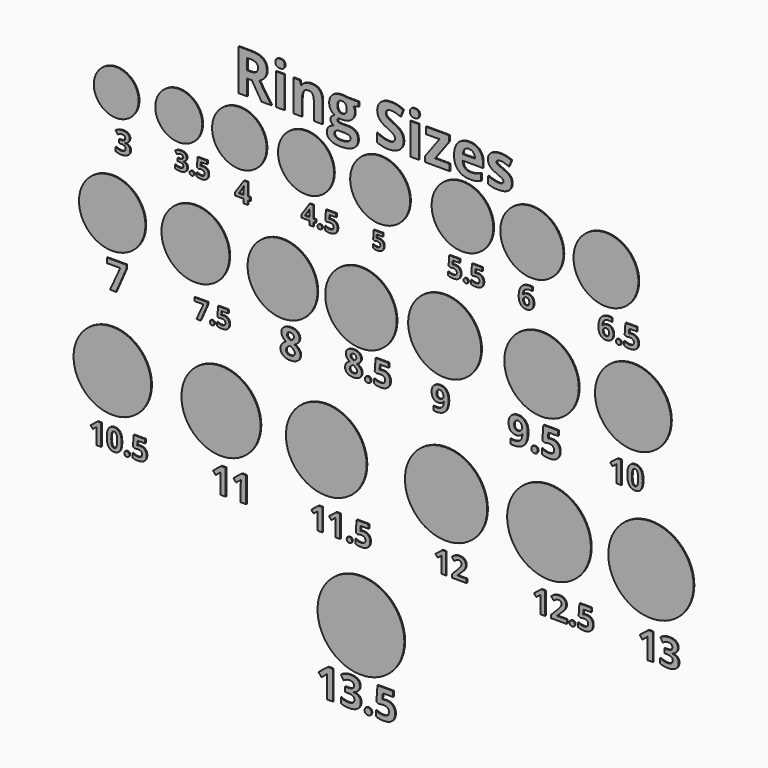
from build123d import *

# Parameters (mm, degrees)
F0_R           = 5.8371680151
F8_DEPTH       = 0.254
F0_R_2         = 6.1199922199
F0_R_3         = 7.0989140275
F0_R_4         = 7.291492477
F0_R_5         = 7.8
F1_R           = 8.0243902439
F1_R_2         = 8.225
F1_R_3         = 8.45
F1_TEXT_SIZE   = 7.715160696
F1_TEXT_SIZE_2 = 6.496977155
F1_TEXT_SIZE_3 = 7.3090960558
F1_TEXT_SIZE_4 = 6.9030366054
F1_TEXT_SIZE_5 = 6.0909125149
F1_TEXT_SIZE_6 = 7.7151555062
F9_DEPTH       = 0.254
F2_R           = 8.65
F2_R_2         = 8.85
F3_R           = 9.1
F3_R_2         = 9.3
F4_R           = 9.504040404
F4_R_2         = 9.7
F4_TEXT_SIZE   = 9.9162159498
F4_TEXT_SIZE_2 = 6.7430258573
F4_TEXT_SIZE_3 = 10.3128641568
F4_TEXT_SIZE_4 = 8.7262694274
F4_TEXT_SIZE_5 = 8.7262713285
F5_R           = 9.9
F5_TEXT_SIZE   = 8.0965381737
F6_R           = 10.1
F6_R_2         = 10.3
F6_R_3         = 10.5
F6_R_4         = 10.7
F6_R_5         = 10.9
F6_R_6         = 11.1
F6_R_7         = 11.3
F6_TEXT_SIZE   = 7.6917129465
F6_TEXT_SIZE_2 = 9.3110190291
F6_TEXT_SIZE_3 = 8.0965355866
F6_TEXT_SIZE_4 = 8.0965407607
F6_TEXT_SIZE_5 = 9.7158468432
F6_TEXT_SIZE_6 = 10.5254921234
F10_DEPTH      = 0.254
F7_TEXT_SIZE   = 14.9785903179
F11_DEPTH      = 0.254


# Not quite as in the source:
# - Text() gives the source's letters only with a copy of the font that has no kerning and outlines rounded to 1/6400 em; it was checked with that copy


with BuildPart() as f8:
    # F0 (on Front) → F8 (new body)
    with BuildSketch(Plane.XZ):
        with Locations((-63.7036129132, 51.7368838191)):
            Circle(F0_R)
    extrude(amount=F8_DEPTH)


with BuildPart() as f8b:
    # F0 (on Front) → F8, piece 2 (new body)
    with BuildSketch(Plane.XZ):
        with Locations((-47.4188692464, 51.7368838191)):
            Circle(F0_R_2)
    extrude(amount=F8_DEPTH)


with BuildPart() as f8c:
    # F0 (on Front) → F8, piece 3 (new body)
    with BuildSketch(Plane.XZ):
        with Locations((-31.6557335996, 51.7368838191)):
            Circle(F0_R_3)
    extrude(amount=F8_DEPTH)


with BuildPart() as f8d:
    # F0 (on Front) → F8, piece 4 (new body)
    with BuildSketch(Plane.XZ):
        with Locations((-14.2972320278, 51.7368838191)):
            Circle(F0_R_4)
    extrude(amount=F8_DEPTH)


with BuildPart() as f8e:
    # F0 (on Front) → F8, piece 5 (new body)
    with BuildSketch(Plane.XZ):
        with Locations((5.0005266884, 51.7368838191)):
            Circle(F0_R_5)
    extrude(amount=F8_DEPTH)


with BuildPart() as f9:
    # F1 (on Front) → F9 (new body)
    with BuildSketch(Plane.XZ):
        with Locations((26.4269726021, 52.6113137603)):
            Circle(F1_R)
        with Locations((44.5094197899, 52.6113137603)):
            Circle(F1_R_2)
        with Locations((63.7865934914, 52.6113137603)):
            Circle(F1_R_3)
        with Locations((-64.1658629432, 37.9931100235)):
            Text('3', F1_TEXT_SIZE, font='Open Sans', font_style=FontStyle.BOLD, text_align=(TextAlign.LEFT, TextAlign.BOTTOM))
        with Locations((-48.670567057, 39.1625649773)):
            Text('3.5', F1_TEXT_SIZE_2, font='Open Sans', font_style=FontStyle.BOLD, text_align=(TextAlign.LEFT, TextAlign.BOTTOM))
        with Locations((-32.8829083665, 37.1160178741)):
            Text('4', F1_TEXT_SIZE_3, font='Open Sans', font_style=FontStyle.BOLD, text_align=(TextAlign.LEFT, TextAlign.BOTTOM))
        with Locations((-15.6334272472, 37.7007472193)):
            Text('4.5', F1_TEXT_SIZE_4, font='Open Sans', font_style=FontStyle.BOLD, text_align=(TextAlign.LEFT, TextAlign.BOTTOM))
        with Locations((2.7855095265, 37.7007472193)):
            Text('5', F1_TEXT_SIZE_5, font='Open Sans', font_style=FontStyle.BOLD, text_align=(TextAlign.LEFT, TextAlign.BOTTOM))
        with Locations((22.3738989185, 37.7007472193)):
            Text('5.5', F1_TEXT_SIZE_4, font='Open Sans', font_style=FontStyle.BOLD, text_align=(TextAlign.LEFT, TextAlign.BOTTOM))
        with Locations((40.7928359258, 36.8236550698)):
            Text('6', F1_TEXT_SIZE_6, font='Open Sans', font_style=FontStyle.BOLD, text_align=(TextAlign.LEFT, TextAlign.BOTTOM))
        with Locations((61.5506847088, 36.5312885289)):
            Text('6.5', F1_TEXT_SIZE, font='Open Sans', font_style=FontStyle.BOLD, text_align=(TextAlign.LEFT, TextAlign.BOTTOM))
    extrude(amount=F9_DEPTH)


with BuildPart() as f10:
    # F2 (on Front) + F3 (on Front) + F4 (on Front) + F5 (on Front) + F6 (on Front) → F10 (new body)
    with BuildSketch(Plane.XZ):
        with Locations((-64.7544219601, 23.7552467734)):
            Circle(F2_R)
        with Locations((-43.0889738008, 23.7552467734)):
            Circle(F2_R_2)
    with BuildSketch(Plane.XZ):
        with Locations((-20.4131133434, 23.1065114508)):
            Circle(F3_R)
        with Locations((0, 23.1065114508)):
            Circle(F3_R_2)
    with BuildSketch(Plane.XZ):
        with Locations((21.7980570294, 23.7242044372)):
            Circle(F4_R)
        with Locations((47.0187727928, 23.1759268651)):
            Circle(F4_R_2)
        with Locations((-66.4158480186, 6.0407065252)):
            Text('7', F4_TEXT_SIZE, font='Open Sans', font_style=FontStyle.BOLD, text_align=(TextAlign.LEFT, TextAlign.BOTTOM))
        with Locations((-43.5688893904, 6.6118803996)):
            Text('7.5', F4_TEXT_SIZE_2, font='Open Sans', font_style=FontStyle.BOLD, text_align=(TextAlign.LEFT, TextAlign.BOTTOM))
        with Locations((-21.2931023554, 5.1839454854)):
            Text('8', F4_TEXT_SIZE_3, font='Open Sans', font_style=FontStyle.BOLD, text_align=(TextAlign.LEFT, TextAlign.BOTTOM))
        with Locations((-4.4434673558, 6.6118803996)):
            Text('8.5', F4_TEXT_SIZE_4, font='Open Sans', font_style=FontStyle.BOLD, text_align=(TextAlign.LEFT, TextAlign.BOTTOM))
        with Locations((18.1179073008, 5.7551189036)):
            Text('9', F4_TEXT_SIZE_5, font='Open Sans', font_style=FontStyle.BOLD, text_align=(TextAlign.LEFT, TextAlign.BOTTOM))
        with Locations((38.108998838, 4.6127711547)):
            Text('9.5', F4_TEXT_SIZE, font='Open Sans', font_style=FontStyle.BOLD, text_align=(TextAlign.LEFT, TextAlign.BOTTOM))
    with BuildSketch(Plane.XZ):
        with Locations((70.8285272121, 23.4637726098)):
            Circle(F5_R)
        with Locations((64.4160658121, 4.5178690925)):
            Text('10', F5_TEXT_SIZE, font='Open Sans', font_style=FontStyle.BOLD, text_align=(TextAlign.LEFT, TextAlign.BOTTOM))
    with BuildSketch(Plane.XZ):
        with Locations((-64.7075399756, -12.3877050355)):
            Circle(F6_R)
        with Locations((-36.4344269037, -12.3877050355)):
            Circle(F6_R_2)
        with Locations((-9.035738185, -12.3877050355)):
            Circle(F6_R_3)
        with Locations((22.1521314234, -12.3877050355)):
            Circle(F6_R_4)
        with Locations((48.9678680897, -12.3877050355)):
            Circle(F6_R_5)
        with Locations((75.4921287298, -12.3877050355)):
            Circle(F6_R_6)
        with Locations((0, -49.6965572238)):
            Circle(F6_R_7)
        with Locations((-70.8285272121, -30.7506565005)):
            Text('10.5', F6_TEXT_SIZE, font='Open Sans', font_style=FontStyle.BOLD, text_align=(TextAlign.LEFT, TextAlign.BOTTOM))
        with Locations((-39.0577055514, -31.6250808537)):
            Text('11', F6_TEXT_SIZE_2, font='Open Sans', font_style=FontStyle.BOLD, text_align=(TextAlign.LEFT, TextAlign.BOTTOM))
        with Locations((-13.4078683332, -31.6250808537)):
            Text('11.5', F6_TEXT_SIZE_3, font='Open Sans', font_style=FontStyle.BOLD, text_align=(TextAlign.LEFT, TextAlign.BOTTOM))
        with Locations((18.945902586, -31.042130664)):
            Text('12', F6_TEXT_SIZE, font='Open Sans', font_style=FontStyle.BOLD, text_align=(TextAlign.LEFT, TextAlign.BOTTOM))
        with Locations((44.5957370102, -31.9165587425)):
            Text('12.5', F6_TEXT_SIZE_4, font='Open Sans', font_style=FontStyle.BOLD, text_align=(TextAlign.LEFT, TextAlign.BOTTOM))
        with Locations((71.9944238663, -33.3739332855)):
            Text('13', F6_TEXT_SIZE_5, font='Open Sans', font_style=FontStyle.BOLD, text_align=(TextAlign.LEFT, TextAlign.BOTTOM))
        with Locations((-11.6590159014, -69.5168823004)):
            Text('13.5', F6_TEXT_SIZE_6, font='Open Sans', font_style=FontStyle.BOLD, text_align=(TextAlign.LEFT, TextAlign.BOTTOM))
    extrude(amount=F10_DEPTH)


with BuildPart() as f11:
    # F7 (on Front) → F11 (new body)
    with BuildSketch(Plane.XZ):
        with Locations((-33.2281962037, 61.9385279715)):
            Text('Ring Sizes', F7_TEXT_SIZE, font='Open Sans', font_style=FontStyle.BOLD, text_align=(TextAlign.LEFT, TextAlign.BOTTOM))
    extrude(amount=F11_DEPTH)


solid = Compound([f8.part, f8b.part, f8c.part, f8d.part, f8e.part, f9.part, f10.part, f11.part])
